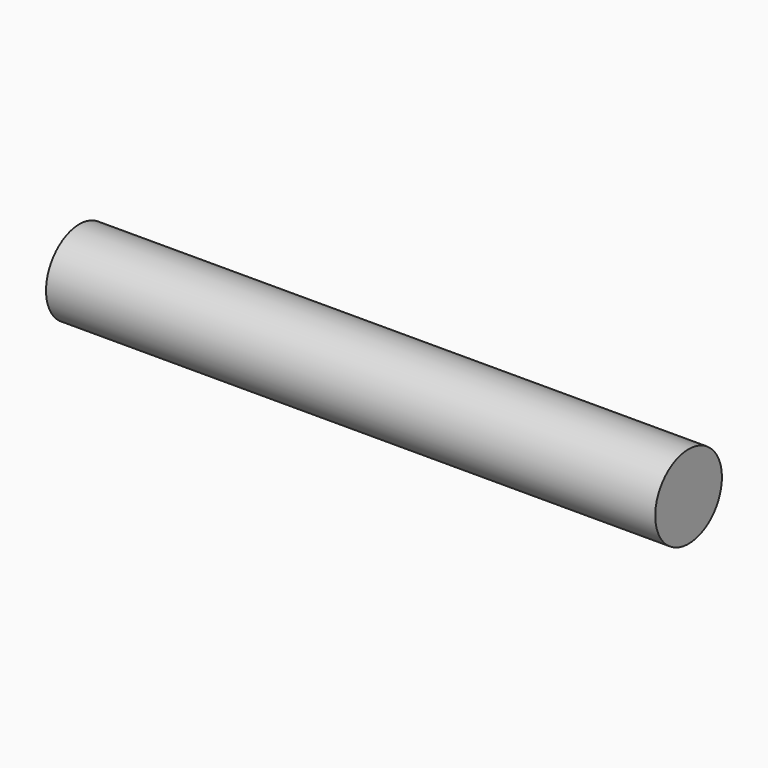
from build123d import *

# Parameters (mm, degrees)
F3_R          = 34.7635785501
F4_DEPTH      = 254
F4_DEPTH_BACK = 254


# Not quite as in the source:
# - the program builds the solid bodies; features that only make, move or delete a surface that nothing else refers to are left out


with BuildPart() as f4:
    # F3 (on face) → F4 (new body, two sides)
    with BuildSketch(Plane.YZ) as f4_sk:
        with Locations((0, 70.0641721487)):
            Circle(F3_R)
    extrude(amount=F4_DEPTH)
    extrude(f4_sk.sketch, amount=-F4_DEPTH_BACK)


solid = f4.part
